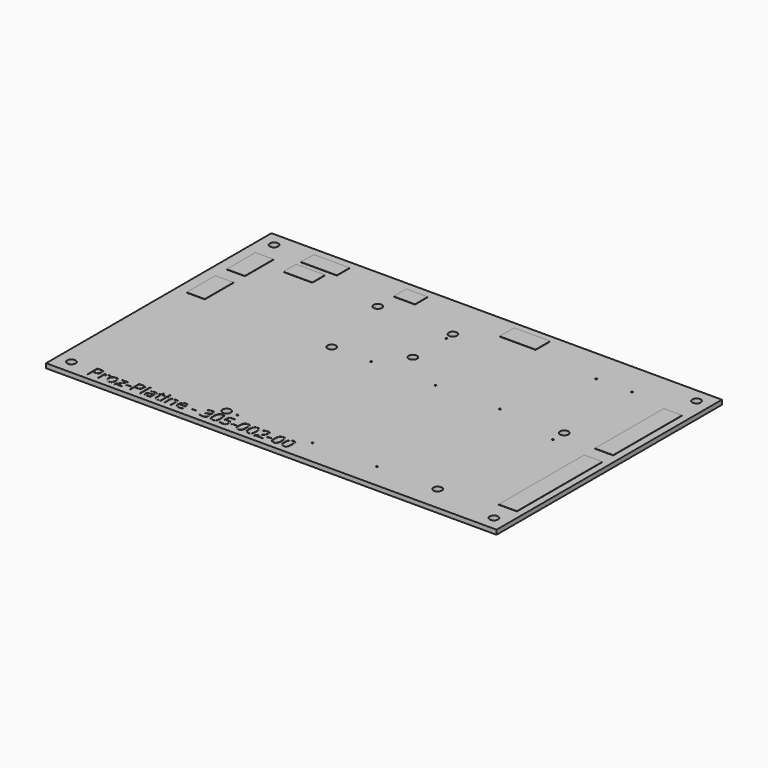
from build123d import *

# Parameters (mm, degrees)
F0_R         = 1.5
F0_R_2       = 0.3
F0_W         = 6.5
F0_H         = 38
F0_H_2       = 12.8
F0_W_2       = 10.3
F0_H_3       = 5.7
F0_W_3       = 12.8
F0_W_4       = 7.6
F0_H_4       = 30.6
F0_H_5       = 6.5
F1_DEPTH     = 1.6
F2_TEXT_SIZE = 6.1743944469
F3_DEPTH     = 0.1
F4_DEPTH     = 0.1


# Not quite as in the source:
# - Text() gives the source's letters only with a copy of the font that has no kerning and outlines rounded to 1/6400 em; it was checked with that copy


with BuildPart() as f1:
    # F0 (on Top) → F1 (new body)
    with BuildSketch(Plane.XY):
        Polygon((-80.0142620787, -49.9771734296), (79.9857314093, -50.0228225004), (80.0142620787, 49.9771734296), (-79.9857314093, 50.0228225004), align=None)
        with Locations((-75.0142620787, -44.9771734296)):
            Circle(F0_R, mode=Mode.SUBTRACT)
        with Locations((-22.9442620787, -41.1671734296)):
            Circle(F0_R, mode=Mode.SUBTRACT)
        with Locations((-19.1342620787, -41.1671734296)):
            Circle(F0_R_2, mode=Mode.SUBTRACT)
        with Locations((7.5357379213, -41.1671734296)):
            Circle(F0_R_2, mode=Mode.SUBTRACT)
        with Locations((30.3957379213, -41.1671734296)):
            Circle(F0_R_2, mode=Mode.SUBTRACT)
        with Locations((51.9857379213, -41.1671734296)):
            Circle(F0_R, mode=Mode.SUBTRACT)
        with Locations((75.0142620787, -44.9771734296)):
            Circle(F0_R, mode=Mode.SUBTRACT)
        with Locations((74.3072302341, -18.9485376179)):
            Rectangle(F0_W, F0_H, mode=Mode.SUBTRACT)
        with Locations((-72.82795012, 13.8352150097)):
            Rectangle(F0_W, F0_H_2, mode=Mode.SUBTRACT)
        with Locations((-24.2142620787, 7.0928265704)):
            Circle(F0_R, mode=Mode.SUBTRACT)
        with Locations((-10.2442620787, 7.0928265704)):
            Circle(F0_R_2, mode=Mode.SUBTRACT)
        with Locations((-2.8345338571, 16.3421019626)):
            Circle(F0_R, mode=Mode.SUBTRACT)
        with Locations((-72.82795012, 31.6185147256)):
            Rectangle(F0_W, F0_H_2, mode=Mode.SUBTRACT)
        with Locations((-57.6909482479, 36.7140769958)):
            Rectangle(F0_W_2, F0_H_3, mode=Mode.SUBTRACT)
        with Locations((-75.0142620787, 44.9771734296)):
            Circle(F0_R, mode=Mode.SUBTRACT)
        with Locations((-56.303486532, 44.317897594)):
            Rectangle(F0_W_3, F0_H_3, mode=Mode.SUBTRACT)
        with Locations((-29.5045338571, 34.1221019626)):
            Circle(F0_R, mode=Mode.SUBTRACT)
        with Locations((-2.6242620787, 31.0071734296)):
            Circle(F0_R_2, mode=Mode.SUBTRACT)
        with Locations((-2.8345338571, 34.1221019626)):
            Circle(F0_R, mode=Mode.SUBTRACT)
        with Locations((-25.9180944413, 44.2578420043)):
            Rectangle(F0_W_4, F0_H_3, mode=Mode.SUBTRACT)
        with Locations((12.6157379213, 7.0928265704)):
            Circle(F0_R_2, mode=Mode.SUBTRACT)
        with Locations((35.4757379213, 7.0928265704)):
            Circle(F0_R_2, mode=Mode.SUBTRACT)
        with Locations((58.3357379213, 2.0128265704)):
            Circle(F0_R_2, mode=Mode.SUBTRACT)
        with Locations((58.3357379213, 7.0928265704)):
            Circle(F0_R, mode=Mode.SUBTRACT)
        with Locations((74.1386115551, 20.2894937247)):
            Rectangle(F0_W, F0_H_4, mode=Mode.SUBTRACT)
        with Locations((14.5959667861, 44.2984439433)):
            Rectangle(F0_W_3, F0_H_5, mode=Mode.SUBTRACT)
        with Locations((44.9950907707, 37.968583405)):
            Circle(F0_R_2, mode=Mode.SUBTRACT)
        with Locations((57.6950907707, 37.968583405)):
            Circle(F0_R_2, mode=Mode.SUBTRACT)
        with Locations((75.0142620787, 44.9771734296)):
            Circle(F0_R, mode=Mode.SUBTRACT)
        with Locations((-72.82795012, 13.8352150097)):
            Rectangle(F0_W, F0_H_2)
        with Locations((-72.82795012, 31.6185147256)):
            Rectangle(F0_W, F0_H_2)
        with Locations((-57.6909482479, 36.7140769958)):
            Rectangle(F0_W_2, F0_H_3)
        with Locations((-56.303486532, 44.317897594)):
            Rectangle(F0_W_3, F0_H_3)
        with Locations((-25.9180944413, 44.2578420043)):
            Rectangle(F0_W_4, F0_H_3)
        with Locations((14.5959667861, 44.2984439433)):
            Rectangle(F0_W_3, F0_H_5)
        with Locations((74.1386115551, 20.2894937247)):
            Rectangle(F0_W, F0_H_4)
        with Locations((74.3072302341, -18.9485376179)):
            Rectangle(F0_W, F0_H)
    extrude(amount=-F1_DEPTH)

    # F2 (on face) → F3 (cut)
    with BuildSketch(Plane.XY):
        with Locations((-67.519094795, -47.9870345443)):
            Text('Proz-Platine - 305-002-00', F2_TEXT_SIZE, font='Open Sans', text_align=(TextAlign.LEFT, TextAlign.BOTTOM))
    extrude(amount=-F3_DEPTH, mode=Mode.SUBTRACT)

    # F0 (on Top) → F4 (join)
    with BuildSketch(Plane.XY):
        with Locations((-72.82795012, 13.8352150097)):
            Rectangle(F0_W, F0_H_2)
        with Locations((-72.82795012, 31.6185147256)):
            Rectangle(F0_W, F0_H_2)
        with Locations((-57.6909482479, 36.7140769958)):
            Rectangle(F0_W_2, F0_H_3)
        with Locations((-56.303486532, 44.317897594)):
            Rectangle(F0_W_3, F0_H_3)
        with Locations((-25.9180944413, 44.2578420043)):
            Rectangle(F0_W_4, F0_H_3)
        with Locations((14.5959667861, 44.2984439433)):
            Rectangle(F0_W_3, F0_H_5)
        with Locations((74.1386115551, 20.2894937247)):
            Rectangle(F0_W, F0_H_4)
        with Locations((74.3072302341, -18.9485376179)):
            Rectangle(F0_W, F0_H)
    extrude(amount=F4_DEPTH)


solid = f1.part
